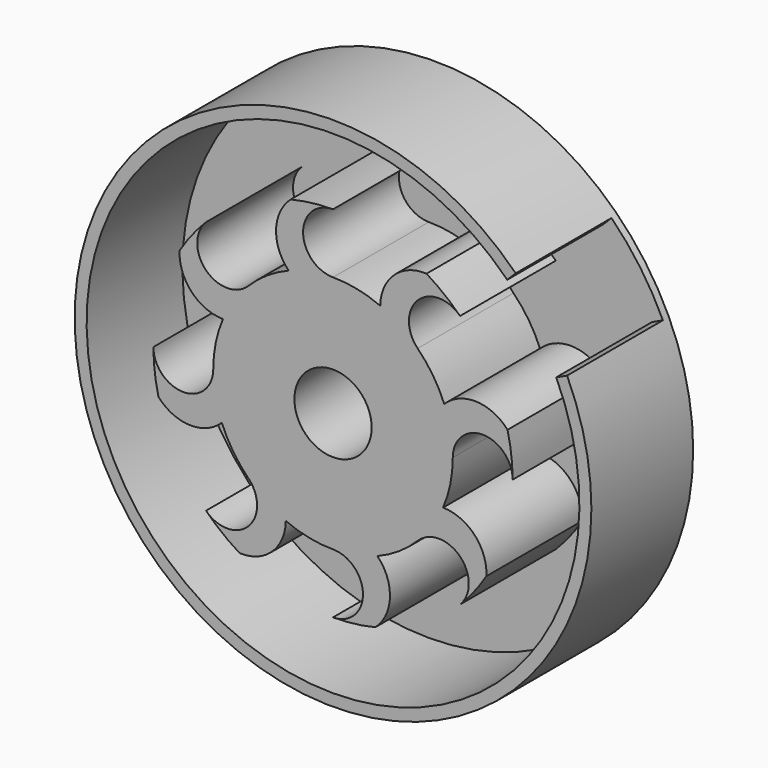
from build123d import *

# Parameters (mm, degrees)
F0_R            = 25.4
F1_DEPTH        = 25.4
F3_DEPTH        = 25.4
F3_COPIES_COUNT = 8
F5_R            = 54.8058055475
F6_DEPTH        = 1.5875
F7_R            = 54.8058055475
F7_R_2          = 52.2658055475
F8_DEPTH        = 25.4
F9_R            = 8.1942220896
F10_DEPTH       = 26.9885
F12_DEPTH       = 25.4


# Not quite as in the source:
# - a pattern or mirror of a feature is missing from the dataset's text; its kind, count and spacing are read off the source's solid


with BuildPart() as f1:
    # F0 (on Front) → F1 (new body)
    with BuildSketch(Plane.XZ):
        Circle(F0_R)
    extrude(amount=F1_DEPTH)

    # F2 (on Front) → F3 (join, through all)
    with BuildSketch(Plane.XZ):
        with BuildLine():
            ThreePointArc((0, 25.4), (-6.35, 31.75), (0, 38.1))
            ThreePointArc((0, 38.1), (-4.5202939278, 37.8308993127), (-8.9767340917, 37.0273985725))
            ThreePointArc((-8.9767340917, 37.0273985725), (-12.0799901727, 30.403051734), (-9.4225081919, 23.5876310674))
            ThreePointArc((-9.4225081919, 23.5876310674), (-4.7976124733, 24.9427928379), (0, 25.4))
        make_face()
    f3 = extrude(amount=F3_DEPTH)

    # F3_copies: F3 ×8 about axis
    f3_copies_axis = Axis((0, 0, 0), (0, 1, 0))
    for i in range(1, F3_COPIES_COUNT):
        add(f3.rotate(f3_copies_axis, i * 360 / F3_COPIES_COUNT))

    # F9 (on face) → F10 (cut, through all)
    with BuildSketch(Plane.XZ.offset(25.4)):
        Circle(F9_R)
    extrude(amount=-F10_DEPTH, mode=Mode.SUBTRACT)


with BuildPart() as f6:
    # F5 (on Front) → F6 (new body)
    with BuildSketch(Plane.XZ):
        Circle(F5_R)
    extrude(amount=-F6_DEPTH)

    # F7 (on face) → F8 (join)
    with BuildSketch(Plane.XZ):
        Circle(F7_R)
        Circle(F7_R_2, mode=Mode.SUBTRACT)
    extrude(amount=F8_DEPTH)

    # F11 (on face) → F12 (cut, through all)
    with BuildSketch(Plane.XZ):
        with BuildLine():
            Line((47.3533162762, 22.1218866098), (49.6545804025, 23.1969602914))
            ThreePointArc((49.6545804025, 23.1969602914), (44.8831995527, 31.4511481447), (38.753556751, 38.753556751))
            Line((38.753556751, 38.753556751), (36.9575055268, 36.9575055268))
            ThreePointArc((36.9575055268, 36.9575055268), (42.8030672433, 29.9935303706), (47.3533162762, 22.1218866098))
        make_face()
    extrude(amount=F12_DEPTH, mode=Mode.SUBTRACT)


solid = Compound([f1.part, f6.part])
